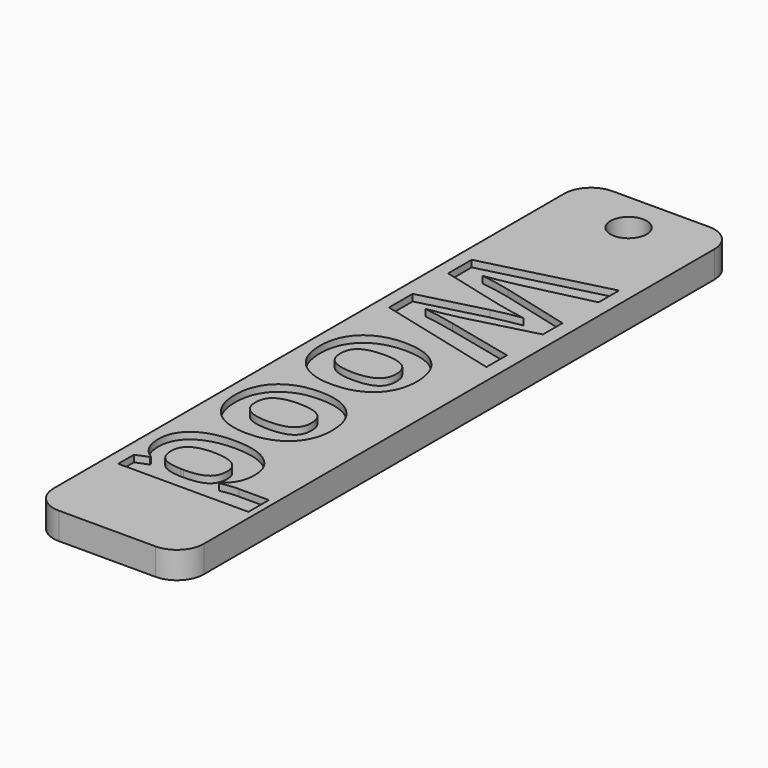
from build123d import *

# Parameters (mm, degrees)
F0_W         = 11.2
F0_H         = 51.6
F0_R         = 1.35
F0_TEXT_SIZE = 12.7777777778
F1_DEPTH     = 2
F2_DEPTH     = 0.5
F3_R         = 2


# Not quite as in the source:
# - Text() gives the source's letters only with a copy of the font that has no kerning and outlines rounded to 1/6400 em; it was checked with that copy


with BuildPart() as f1:
    # F0 (on Top) → F1 (new body)
    with BuildSketch(Plane.XY):
        with Locations((-43.6647401989, 48.8899732466)):
            Rectangle(F0_W, F0_H)
        with BuildLine():
            add(Edge.make_bspline(
                [(-42.8491586016, 37.9478725522), (-43.6667367266, 37.53658783), (-44.7648270044, 37.53658783)],
                knots=[0, 0, 0, 1, 1, 1], degree=2))
            add(Edge.make_bspline(
                [(-44.7648270044, 37.53658783), (-46.4678651989, 37.53658783), (-47.4291933239, 38.43502533)],
                knots=[0, 0, 0, 1, 1, 1], degree=2))
            add(Edge.make_bspline(
                [(-47.4291933239, 38.43502533), (-48.3905214489, 39.33346283), (-48.3905214489, 40.9366746355)],
                knots=[0, 0, 0, 1, 1, 1], degree=2))
            add(Edge.make_bspline(
                [(-48.3905214489, 40.9366746355), (-48.3905214489, 41.9409281077), (-47.9502870739, 42.7085930383)],
                knots=[0, 0, 0, 1, 1, 1], degree=2))
            add(Edge.make_bspline(
                [(-47.9502870739, 42.7085930383), (-47.5100526989, 43.4762579688), (-46.6864849905, 43.8875426911)],
                knots=[0, 0, 0, 1, 1, 1], degree=2))
            add(Edge.make_bspline(
                [(-46.6864849905, 43.8875426911), (-45.8629172822, 44.2988274133), (-44.7648270044, 44.2988274133)],
                knots=[0, 0, 0, 1, 1, 1], degree=2))
            add(Edge.make_bspline(
                [(-44.7648270044, 44.2988274133), (-43.0557992266, 44.2988274133), (-42.1074485322, 43.4073777605)],
                knots=[0, 0, 0, 1, 1, 1], degree=2))
            add(Edge.make_bspline(
                [(-42.1074485322, 43.4073777605), (-41.1590978377, 42.5159281077), (-41.1590978377, 40.8987406077)],
                knots=[0, 0, 0, 1, 1, 1], degree=2))
            add(Edge.make_bspline(
                [(-41.1590978377, 40.8987406077), (-41.1590978377, 39.8944871355), (-41.5953391572, 39.126822205)],
                knots=[0, 0, 0, 1, 1, 1], degree=2))
            add(Edge.make_bspline(
                [(-41.5953391572, 39.126822205), (-42.0315804766, 38.3591572744), (-42.8491586016, 37.9478725522)],
                knots=[0, 0, 0, 1, 1, 1], degree=2))
        make_face(mode=Mode.SUBTRACT)
        with BuildLine():
            add(Edge.make_bspline(
                [(-42.8491586016, 45.8601121355), (-43.6667367266, 45.4488274133), (-44.7648270044, 45.4488274133)],
                knots=[0, 0, 0, 1, 1, 1], degree=2))
            add(Edge.make_bspline(
                [(-44.7648270044, 45.4488274133), (-46.4678651989, 45.4488274133), (-47.4291933239, 46.3472649133)],
                knots=[0, 0, 0, 1, 1, 1], degree=2))
            add(Edge.make_bspline(
                [(-47.4291933239, 46.3472649133), (-48.3905214489, 47.2457024133), (-48.3905214489, 48.8489142188)],
                knots=[0, 0, 0, 1, 1, 1], degree=2))
            add(Edge.make_bspline(
                [(-48.3905214489, 48.8489142188), (-48.3905214489, 49.8531676911), (-47.9502870739, 50.6208326216)],
                knots=[0, 0, 0, 1, 1, 1], degree=2))
            add(Edge.make_bspline(
                [(-47.9502870739, 50.6208326216), (-47.5100526989, 51.3884975522), (-46.6864849905, 51.7997822744)],
                knots=[0, 0, 0, 1, 1, 1], degree=2))
            add(Edge.make_bspline(
                [(-46.6864849905, 51.7997822744), (-45.8629172822, 52.2110669966), (-44.7648270044, 52.2110669966)],
                knots=[0, 0, 0, 1, 1, 1], degree=2))
            add(Edge.make_bspline(
                [(-44.7648270044, 52.2110669966), (-43.0557992266, 52.2110669966), (-42.1074485322, 51.3196173438)],
                knots=[0, 0, 0, 1, 1, 1], degree=2))
            add(Edge.make_bspline(
                [(-42.1074485322, 51.3196173438), (-41.1590978377, 50.4281676911), (-41.1590978377, 48.8109801911)],
                knots=[0, 0, 0, 1, 1, 1], degree=2))
            add(Edge.make_bspline(
                [(-41.1590978377, 48.8109801911), (-41.1590978377, 47.8067267188), (-41.5953391572, 47.0390617883)],
                knots=[0, 0, 0, 1, 1, 1], degree=2))
            add(Edge.make_bspline(
                [(-41.5953391572, 47.0390617883), (-42.0315804766, 46.2713968577), (-42.8491586016, 45.8601121355)],
                knots=[0, 0, 0, 1, 1, 1], degree=2))
        make_face(mode=Mode.SUBTRACT)
        with BuildLine():
            add(Edge.make_bspline(
                [(-47.3603131155, 31.7766051911), (-48.3905214489, 32.4254767188), (-48.3905214489, 33.7551642188)],
                knots=[0, 0, 0, 1, 1, 1], degree=2))
            add(Edge.make_bspline(
                [(-48.3905214489, 33.7551642188), (-48.3905214489, 34.9830288022), (-47.4351829072, 35.6848083161)],
                knots=[0, 0, 0, 1, 1, 1], degree=2))
            add(Edge.make_bspline(
                [(-47.4351829072, 35.6848083161), (-46.4798443655, 36.38658783), (-44.7887853377, 36.38658783)],
                knots=[0, 0, 0, 1, 1, 1], degree=2))
            add(Edge.make_bspline(
                [(-44.7887853377, 36.38658783), (-43.0737679766, 36.38658783), (-42.1164329072, 35.6728291494)],
                knots=[0, 0, 0, 1, 1, 1], degree=2))
            add(Edge.make_bspline(
                [(-42.1164329072, 35.6728291494), (-41.1590978377, 34.9590704688), (-41.1590978377, 33.7052510244)],
                knots=[0, 0, 0, 1, 1, 1], degree=2))
            add(Edge.make_bspline(
                [(-41.1590978377, 33.7052510244), (-41.1590978377, 32.3875426911), (-42.18132006, 31.6947475522)],
                knots=[0, 0, 0, 1, 1, 1], degree=2))
            Line((-42.18132006, 31.6947475522), (-42.18132006, 31.6328551911))
            add(Edge.make_bspline(
                [(-42.18132006, 31.6328551911), (-41.4006776989, 31.7766051911), (-40.7897401989, 31.7766051911)],
                knots=[0, 0, 0, 1, 1, 1], degree=2))
            Line((-40.7897401989, 31.7766051911), (-38.5556256155, 31.7766051911))
            Line((-38.5556256155, 31.7766051911), (-38.5556256155, 29.8679246355))
            Line((-38.5556256155, 29.8679246355), (-48.2647401989, 29.8679246355))
            Line((-48.2647401989, 29.8679246355), (-48.2647401989, 31.3273864411))
            Line((-48.2647401989, 31.3273864411), (-47.3603131155, 31.6947475522))
            Line((-47.3603131155, 31.6947475522), (-47.3603131155, 31.7766051911))
        make_face(mode=Mode.SUBTRACT)
        with BuildLine():
            Line((-39.1426047822, 52.7860669966), (-48.2647401989, 55.1080288022))
            Line((-48.2647401989, 55.1080288022), (-48.2647401989, 57.3101989411))
            Line((-48.2647401989, 57.3101989411), (-43.4730735322, 58.5460496355))
            add(Edge.make_bspline(
                [(-43.4730735322, 58.5460496355), (-43.2175179766, 58.61393158), (-42.4159120739, 58.7796433855)],
                knots=[0, 0, 0, 1, 1, 1], degree=2))
            add(Edge.make_bspline(
                [(-42.4159120739, 58.7796433855), (-41.6143061711, 58.9453551911), (-41.3387853377, 58.9693135244)],
                knots=[0, 0, 0, 1, 1, 1], degree=2))
            add(Edge.make_bspline(
                [(-41.3387853377, 58.9693135244), (-41.6761985322, 59.0072475522), (-42.4219016572, 59.1569871355)],
                knots=[0, 0, 0, 1, 1, 1], degree=2))
            add(Edge.make_bspline(
                [(-42.4219016572, 59.1569871355), (-43.1676047822, 59.3067267188), (-43.4850526989, 59.3885843577)],
                knots=[0, 0, 0, 1, 1, 1], degree=2))
            Line((-43.4850526989, 59.3885843577), (-48.2647401989, 60.6164489411))
            Line((-48.2647401989, 60.6164489411), (-48.2647401989, 62.8126294966))
            Line((-48.2647401989, 62.8126294966), (-39.1426047822, 65.1405808855))
            Line((-39.1426047822, 65.1405808855), (-39.1426047822, 63.2378899133))
            Line((-39.1426047822, 63.2378899133), (-44.12194506, 62.0699211633))
            add(Edge.make_bspline(
                [(-44.12194506, 62.0699211633), (-45.5015457544, 61.7644524133), (-46.51178881, 61.6286885244)],
                knots=[0, 0, 0, 1, 1, 1], degree=2))
            add(Edge.make_bspline(
                [(-46.51178881, 61.6286885244), (-46.1564068655, 61.5907544966), (-45.4107037405, 61.4559888716)],
                knots=[0, 0, 0, 1, 1, 1], degree=2))
            add(Edge.make_bspline(
                [(-45.4107037405, 61.4559888716), (-44.6650006155, 61.3212232466), (-44.2537158933, 61.2034281077)],
                knots=[0, 0, 0, 1, 1, 1], degree=2))
            Line((-44.2537158933, 61.2034281077), (-39.1426047822, 59.8737406077))
            Line((-39.1426047822, 59.8737406077), (-39.1426047822, 58.0469176911))
            Line((-39.1426047822, 58.0469176911), (-44.2537158933, 56.7172301911))
            add(Edge.make_bspline(
                [(-44.2537158933, 56.7172301911), (-44.5951221433, 56.6293829688), (-45.3008947127, 56.4986103994)],
                knots=[0, 0, 0, 1, 1, 1], degree=2))
            add(Edge.make_bspline(
                [(-45.3008947127, 56.4986103994), (-46.0066672822, 56.36783783), (-46.51178881, 56.2999558855)],
                knots=[0, 0, 0, 1, 1, 1], degree=2))
            add(Edge.make_bspline(
                [(-46.51178881, 56.2999558855), (-46.0246360322, 56.2380635244), (-45.2978999211, 56.1003031077)],
                knots=[0, 0, 0, 1, 1, 1], degree=2))
            add(Edge.make_bspline(
                [(-45.2978999211, 56.1003031077), (-44.57116381, 55.9625426911), (-44.12194506, 55.8507371355)],
                knots=[0, 0, 0, 1, 1, 1], degree=2))
            Line((-44.12194506, 55.8507371355), (-39.1426047822, 54.6907544966))
            Line((-39.1426047822, 54.6907544966), (-39.1426047822, 52.7860669966))
        make_face(mode=Mode.SUBTRACT)
        with Locations((-43.6647401989, 71.6899732466)):
            Circle(F0_R, mode=Mode.SUBTRACT)
        with Locations(Location((-48.2647401989, 65.1405808855), (0, 0, -90))):
            Text('Wood', F0_TEXT_SIZE, font='Open Sans', font_style=FontStyle.BOLD, text_align=(TextAlign.LEFT, TextAlign.BOTTOM))
        with BuildLine():
            add(Edge.make_bspline(
                [(-43.2075353377, 42.0227857466), (-43.7226395044, 42.3601989411), (-44.7648270044, 42.3601989411)],
                knots=[0, 0, 0, 1, 1, 1], degree=2))
            add(Edge.make_bspline(
                [(-44.7648270044, 42.3601989411), (-45.8010249211, 42.3601989411), (-46.3311030461, 42.019790955)],
                knots=[0, 0, 0, 1, 1, 1], degree=2))
            add(Edge.make_bspline(
                [(-46.3311030461, 42.019790955), (-46.8611811711, 41.6793829688), (-46.8611811711, 40.9127163022)],
                knots=[0, 0, 0, 1, 1, 1], degree=2))
            add(Edge.make_bspline(
                [(-46.8611811711, 40.9127163022), (-46.8611811711, 40.1500426911), (-46.3340978377, 39.8166225522)],
                knots=[0, 0, 0, 1, 1, 1], degree=2))
            add(Edge.make_bspline(
                [(-46.3340978377, 39.8166225522), (-45.8070145044, 39.4832024133), (-44.7648270044, 39.4832024133)],
                knots=[0, 0, 0, 1, 1, 1], degree=2))
            add(Edge.make_bspline(
                [(-44.7648270044, 39.4832024133), (-43.7286290877, 39.4832024133), (-43.2105301294, 39.8196173438)],
                knots=[0, 0, 0, 1, 1, 1], degree=2))
            add(Edge.make_bspline(
                [(-43.2105301294, 39.8196173438), (-42.6924311711, 40.1560322744), (-42.6924311711, 40.9246954688)],
                knots=[0, 0, 0, 1, 1, 1], degree=2))
            add(Edge.make_bspline(
                [(-42.6924311711, 40.9246954688), (-42.6924311711, 41.6853725522), (-43.2075353377, 42.0227857466)],
                knots=[0, 0, 0, 1, 1, 1], degree=2))
        make_face()
        with BuildLine():
            add(Edge.make_bspline(
                [(-43.2075353377, 49.93502533), (-43.7226395044, 50.2724385244), (-44.7648270044, 50.2724385244)],
                knots=[0, 0, 0, 1, 1, 1], degree=2))
            add(Edge.make_bspline(
                [(-44.7648270044, 50.2724385244), (-45.8010249211, 50.2724385244), (-46.3311030461, 49.9320305383)],
                knots=[0, 0, 0, 1, 1, 1], degree=2))
            add(Edge.make_bspline(
                [(-46.3311030461, 49.9320305383), (-46.8611811711, 49.5916225522), (-46.8611811711, 48.8249558855)],
                knots=[0, 0, 0, 1, 1, 1], degree=2))
            add(Edge.make_bspline(
                [(-46.8611811711, 48.8249558855), (-46.8611811711, 48.0622822744), (-46.3340978377, 47.7288621355)],
                knots=[0, 0, 0, 1, 1, 1], degree=2))
            add(Edge.make_bspline(
                [(-46.3340978377, 47.7288621355), (-45.8070145044, 47.3954419966), (-44.7648270044, 47.3954419966)],
                knots=[0, 0, 0, 1, 1, 1], degree=2))
            add(Edge.make_bspline(
                [(-44.7648270044, 47.3954419966), (-43.7286290877, 47.3954419966), (-43.2105301294, 47.7318569272)],
                knots=[0, 0, 0, 1, 1, 1], degree=2))
            add(Edge.make_bspline(
                [(-43.2105301294, 47.7318569272), (-42.6924311711, 48.0682718577), (-42.6924311711, 48.8369350522)],
                knots=[0, 0, 0, 1, 1, 1], degree=2))
            add(Edge.make_bspline(
                [(-42.6924311711, 48.8369350522), (-42.6924311711, 49.5976121355), (-43.2075353377, 49.93502533)],
                knots=[0, 0, 0, 1, 1, 1], degree=2))
        make_face()
        with BuildLine():
            add(Edge.make_bspline(
                [(-46.3580561711, 34.10455658), (-46.8731603377, 33.7491746355), (-46.8731603377, 33.0863274133)],
                knots=[0, 0, 0, 1, 1, 1], degree=2))
            add(Edge.make_bspline(
                [(-46.8731603377, 33.0863274133), (-46.8731603377, 32.3575947744), (-46.448898185, 32.0171867883)],
                knots=[0, 0, 0, 1, 1, 1], degree=2))
            add(Edge.make_bspline(
                [(-46.448898185, 32.0171867883), (-46.0246360322, 31.6767788022), (-45.0084033933, 31.6448343577)],
                knots=[0, 0, 0, 1, 1, 1], degree=2))
            Line((-45.0084033933, 31.6448343577), (-44.8027610322, 31.6448343577))
            add(Edge.make_bspline(
                [(-44.8027610322, 31.6448343577), (-43.6787158933, 31.6448343577), (-43.1925613794, 31.9912319272)],
                knots=[0, 0, 0, 1, 1, 1], degree=2))
            add(Edge.make_bspline(
                [(-43.1925613794, 31.9912319272), (-42.7064068655, 32.3376294966), (-42.7064068655, 33.1182718577)],
                knots=[0, 0, 0, 1, 1, 1], degree=2))
            add(Edge.make_bspline(
                [(-42.7064068655, 33.1182718577), (-42.7064068655, 33.7551642188), (-43.2454693655, 34.1075513716)],
                knots=[0, 0, 0, 1, 1, 1], degree=2))
            add(Edge.make_bspline(
                [(-43.2454693655, 34.1075513716), (-43.7845318655, 34.4599385244), (-44.8147401989, 34.4599385244)],
                knots=[0, 0, 0, 1, 1, 1], degree=2))
            add(Edge.make_bspline(
                [(-44.8147401989, 34.4599385244), (-45.8429520044, 34.4599385244), (-46.3580561711, 34.10455658)],
                knots=[0, 0, 0, 1, 1, 1], degree=2))
        make_face()
    extrude(amount=-F1_DEPTH)

    # F0 (on Top) → F2 (cut)
    with BuildSketch(Plane.XY):
        with Locations(Location((-48.2647401989, 65.1405808855), (0, 0, -90))):
            Text('Wood', F0_TEXT_SIZE, font='Open Sans', font_style=FontStyle.BOLD, text_align=(TextAlign.LEFT, TextAlign.BOTTOM))
    extrude(amount=-F2_DEPTH, mode=Mode.SUBTRACT)

    # F3
    f3_edges = [f1.edges().sort_by_distance(p)[0] for p in [
        (-49.26474, 74.689973, -1),
        (-38.06474, 74.689973, -1),
        (-38.06474, 23.089973, -1),
        (-49.26474, 23.089973, -1),
    ]]
    fillet(f3_edges, radius=F3_R)


solid = f1.part
